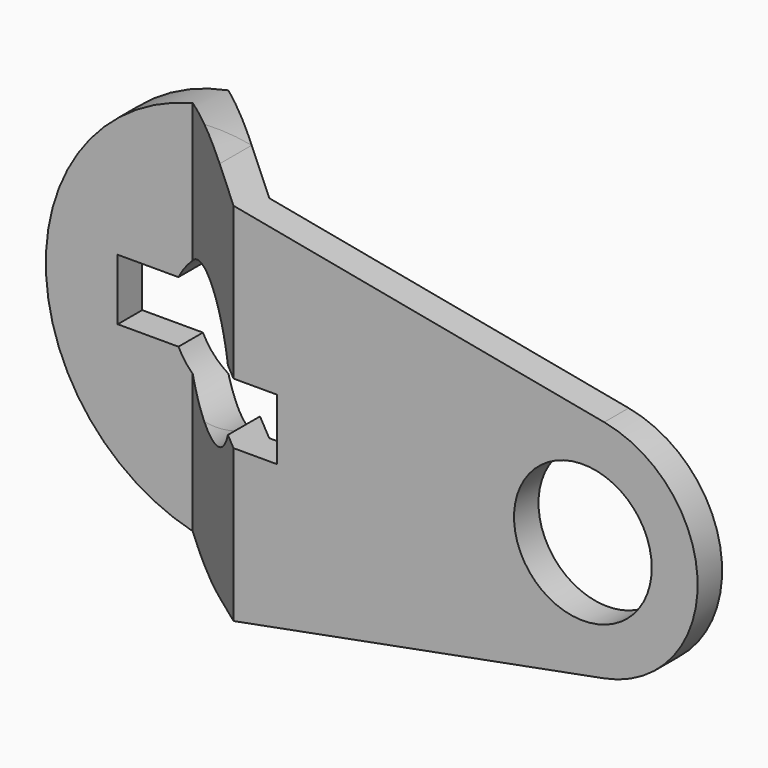
from build123d import *
from build123d import SkipClean  # not in build123d's __all__

# Parameters (mm, degrees)
F0_R     = 22.5
F1_DEPTH = 25
F2_DEPTH = 20
F4_START = 63.501
F4_DEPTH = 127.002


with BuildPart() as f1:
    # F0 (on Front) → F1 (new body)
    with BuildSketch(Plane.XZ):
        with BuildLine():
            ThreePointArc((-51.7071428571, -62.3953405344), (-14.6067671933, -40.5179193162), (0, 0))
            ThreePointArc((0, 0), (-14.6067671933, 40.5179193162), (-51.7071428571, 62.3953405344))
            ThreePointArc((-51.7071428571, 62.3953405344), (-127, 0), (-51.7071428571, -62.3953405344))
        make_face()
        with BuildLine():
            ThreePointArc((-83.6556443707, 10), (-63.5, 22.5), (-43.3443556293, 10))
            Line((-43.3443556293, 10), (-23.5, 10))
            Line((-23.5, 10), (-23.5, -10))
            Line((-23.5, -10), (-43.3443556293, -10))
            ThreePointArc((-43.3443556293, -10), (-63.5, -22.5), (-83.6556443707, -10))
            Line((-83.6556443707, -10), (-103.5, -10))
            Line((-103.5, -10), (-103.5, 10))
            Line((-103.5, 10), (-83.6556443707, 10))
        make_face(mode=Mode.SUBTRACT)
        with BuildLine():
            ThreePointArc((-51.7071428571, 62.3953405344), (-14.6067671933, 40.5179193162), (0, 0))
            ThreePointArc((0, 0), (-14.6067671933, -40.5179193162), (-51.7071428571, -62.3953405344))
            Line((-51.7071428571, -62.3953405344), (83.4642857143, -36.8476420479))
            ThreePointArc((83.4642857143, -36.8476420479), (39, 0), (83.4642857143, 36.8476420479))
            Line((83.4642857143, 36.8476420479), (-51.7071428571, 62.3953405344))
        make_face()
        with BuildLine():
            ThreePointArc((114, 0), (105.3739563819, 23.927905108), (83.4642857143, 36.8476420479))
            ThreePointArc((83.4642857143, 36.8476420479), (39, 0), (83.4642857143, -36.8476420479))
            ThreePointArc((83.4642857143, -36.8476420479), (105.3739563819, -23.927905108), (114, 0))
        make_face()
        with Locations((76.5, 0)):
            Circle(F0_R, mode=Mode.SUBTRACT)
    extrude(amount=F1_DEPTH)

    # F0 (on Front) → F2 (join)
    with BuildSketch(Plane.XZ):
        with BuildLine():
            ThreePointArc((-51.7071428571, -62.3953405344), (-14.6067671933, -40.5179193162), (0, 0))
            ThreePointArc((0, 0), (-14.6067671933, 40.5179193162), (-51.7071428571, 62.3953405344))
            ThreePointArc((-51.7071428571, 62.3953405344), (-127, 0), (-51.7071428571, -62.3953405344))
        make_face()
        with BuildLine():
            ThreePointArc((-83.6556443707, 10), (-63.5, 22.5), (-43.3443556293, 10))
            Line((-43.3443556293, 10), (-23.5, 10))
            Line((-23.5, 10), (-23.5, -10))
            Line((-23.5, -10), (-43.3443556293, -10))
            ThreePointArc((-43.3443556293, -10), (-63.5, -22.5), (-83.6556443707, -10))
            Line((-83.6556443707, -10), (-103.5, -10))
            Line((-103.5, -10), (-103.5, 10))
            Line((-103.5, 10), (-83.6556443707, 10))
        make_face(mode=Mode.SUBTRACT)
    with SkipClean():  # cleaning this boolean's faces spoils the solid; the shape is the same uncleaned
        extrude(amount=-F2_DEPTH)

    # F3 (on Top) → F4 (intersect)
    with BuildSketch(Plane.XY.offset(F4_START)):
        Polygon((-75.3271334507, 20), (-158.5341542959, 20), (-158.5341542959, 10), (-78.9921499119, 10), (-37.6571663732, -25), (141.5535062551, -25), (141.5535062551, -15), (-33.9921499119, -15), align=None)
    with SkipClean():  # cleaning this boolean's faces spoils the solid; the shape is the same uncleaned
        extrude(amount=-F4_DEPTH, mode=Mode.INTERSECT)


solid = f1.part
